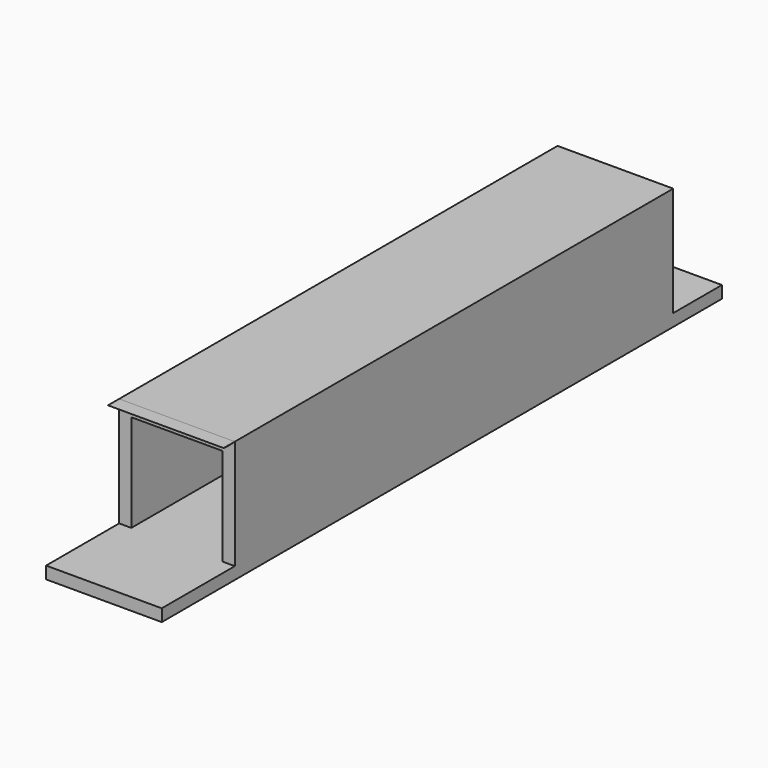
from build123d import *

# Parameters (mm, degrees)
F0_W     = 10
F0_H     = 2
F0_W_2   = 15
F1_DEPTH = 9.5
F2_T     = -2


# Not quite as in the source:
# - a shell that OpenCascade refuses in one call is made with other operations: the cavity is built on its own and cut out


with BuildPart() as f1:
    # F0 (on Right) → F1 (new body, symmetric)
    with BuildSketch(Plane.YZ):
        Polygon((45, 10), (-45, 10), (-45, 8), (-45, 0), (-45, -8), (-45, -10), (45, -10), (45, -8), align=None)
        with Locations((50, -9)):
            Rectangle(F0_W, F0_H)
        with Locations((-52.5, -9)):
            Rectangle(F0_W_2, F0_H)
    extrude(amount=F1_DEPTH, both=True)

    # F2: a shell. OpenCascade refuses it in one call, so the cavity is built on its own and cut out:
    # the body offset inwards by the wall thickness, plus a prism from it out through each open face.
    f2_core = offset(f1.part, amount=F2_T, kind=Kind.INTERSECTION, mode=Mode.PRIVATE)
    f2_exits = [f2_core.faces().sort_by_distance(p)[0] for p in [
        (0, -43, 0),
        (0, 43, 0),
    ]]
    add(f2_core, mode=Mode.SUBTRACT)
    extrude(f2_exits, amount=-F2_T, mode=Mode.SUBTRACT)


with BuildPart() as f1b:
    # F0 (on Right) → F1, piece 2 (new body, symmetric)
    with BuildSketch(Plane.YZ):
        with BuildLine():
            ThreePointArc((-47.2923916416, 10), (-46.1461958208, 9.938642669), (-45, 10))
            Line((-45, 10), (-47.2923916416, 10))
        make_face()
    extrude(amount=F1_DEPTH, both=True)


solid = Compound([f1.part, f1b.part])
